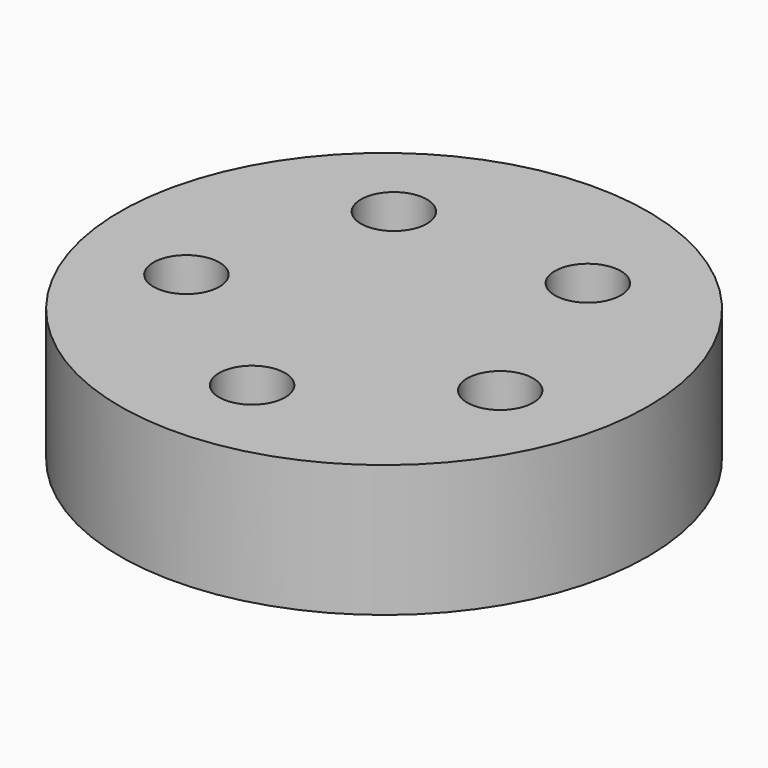
from build123d import *

# Parameters (mm, degrees)
F0_R            = 50.8
F1_DEPTH        = 25.4
F2_R            = 6.35
F4_DEPTH        = 25.401
F4_COPIES_COUNT = 5


# Not quite as in the source:
# - a pattern or mirror of a feature is missing from the dataset's text; its kind, count and spacing are read off the source's solid


with BuildPart() as f1:
    # F0 (on Top) → F1 (new body)
    with BuildSketch(Plane.XY):
        Circle(F0_R)
    extrude(amount=F1_DEPTH)

    # F2 (on face) → F4 (cut, through all)
    with BuildSketch(Plane.XY.offset(25.4)):
        with Locations((0, -31.75)):
            Circle(F2_R)
    f4 = extrude(amount=-F4_DEPTH, mode=Mode.SUBTRACT)

    # F4_copies: F4 ×5 about axis
    f4_copies_axis = Axis((0, 0, 0), (0, 0, 1))
    for i in range(1, F4_COPIES_COUNT):
        add(f4.rotate(f4_copies_axis, i * 360 / F4_COPIES_COUNT), mode=Mode.SUBTRACT)


solid = f1.part
